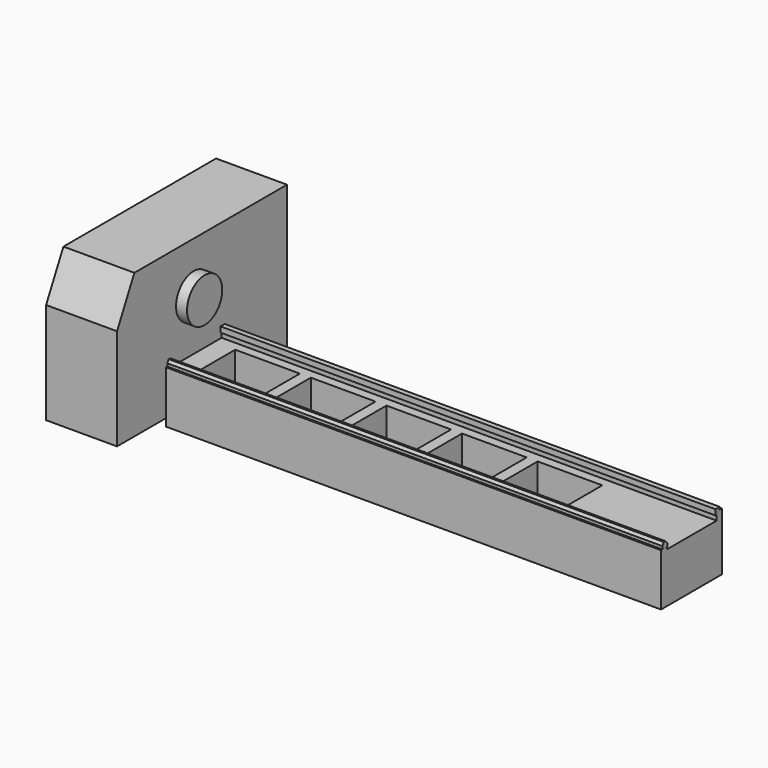
from build123d import *

# Parameters (mm, degrees)
F0_R     = 20
F1_DEPTH = 64.5
F0_W     = 69.1690184176
F0_H     = 6.8107743772
F2_DEPTH = 450
F3_W     = 402.7799852192
F3_H     = 51.0824993253
F4_DEPTH = 15
F5_W     = 58.800008148
F5_H     = 40.4249988496
F6_DEPTH = 40
F7_DEPTH = 450
F8_DEPTH = 10


# Not quite as in the source:
# - a feature names something its author has since deleted; it is built from what else it names


with BuildPart() as f1:
    # F0 (on Right) → F1 (new body)
    with BuildSketch(Plane.YZ):
        Polygon((-87.0358720422, 23.9922005967), (-87.0358720422, -68.190318747), (-31.3871668349, -68.190318747), (-31.3871668349, -27.5489028139), (-29.7969614784, -27.5489028139), (-29.7969614784, -24.9276731835), (-28.2796746202, -22.2527954323), (-26.482412375, -22.2527954323), (-24.0200519564, -24.9276731835), (-24.0200519564, -27.412929792), (-24.6065106683, -27.412929792), (-24.6065106683, -29.5631634037), (31.7927369408, -29.5631634037), (31.7927369408, -24.8985635082), (30.5205726556, -24.8985635082), (30.5205726556, -19.9159244041), (35.2954028477, -19.9159244041), (35.2954028477, -22.2527954323), (37.7818515827, -22.2527954323), (37.7818515827, -68.190318747), (106.1147302389, -68.190318747), (106.1147302389, 62.7493981556), (-67.339591682, 62.7493981556), align=None)
        with Locations((0, 16.7493981556)):
            Circle(F0_R, mode=Mode.SUBTRACT)
        Polygon((-31.3871668349, -27.5489028139), (-31.3871668349, -68.190318747), (37.7818515827, -68.190318747), (37.7818515827, -22.2527954323), (35.2954028477, -22.2527954323), (31.7927369408, -24.8985635082), (31.7927369408, -29.5631634037), (-24.6065106683, -29.5631634037), (-24.6065106683, -27.412929792), (-29.7969614784, -27.5489028139), align=None)
        with Locations((0, 16.7493981556)):
            Circle(F0_R)
        Polygon((-29.7969614784, -24.9276731835), (-29.7969614784, -27.5489028139), (-24.6065106683, -27.412929792), (-24.0200519564, -27.412929792), (-24.0200519564, -24.9276731835), (-26.482412375, -22.2527954323), (-28.2796746202, -22.2527954323), align=None)
        Polygon((31.7927369408, -24.8985635082), (35.2954028477, -22.2527954323), (35.2954028477, -19.9159244041), (30.5205726556, -19.9159244041), (30.5205726556, -24.8985635082), align=None)
    extrude(amount=-F1_DEPTH)


with BuildPart() as f2:
    # F0 (on Right) → F2 (new body)
    with BuildSketch(Plane.YZ):
        with Locations((3.1973423739, -71.5957059356)):
            Rectangle(F0_W, F0_H)
        Polygon((-31.3871668349, -27.5489028139), (-31.3871668349, -68.190318747), (37.7818515827, -68.190318747), (37.7818515827, -22.2527954323), (35.2954028477, -22.2527954323), (31.7927369408, -24.8985635082), (31.7927369408, -29.5631634037), (-24.6065106683, -29.5631634037), (-24.6065106683, -27.412929792), (-29.7969614784, -27.5489028139), align=None)
    extrude(amount=F2_DEPTH)

    # F3 (on face) → F4 (cut)
    with BuildSketch(Plane(origin=(0, 0, -75.0010931242), x_dir=(1, 0, 0), z_dir=(0, 0, -1))):
        with Locations((225.1687403768, -2.7406793088)):
            Rectangle(F3_W, F3_H)
    extrude(amount=-F4_DEPTH, mode=Mode.SUBTRACT)

    # F5 (on face) → F6 (cut)
    with BuildSketch(Plane.XY.offset(-29.5631634037)):
        with Locations((48.4012458473, 3.2919291407)):
            Rectangle(F5_W, F5_H)
        with Locations((323.291266337, 3.2919291407)):
            Rectangle(F5_W, F5_H)
        with Locations((117.1237509698, 3.2919291407)):
            Rectangle(F5_W, F5_H)
        with Locations((185.8462560922, 3.2919291407)):
            Rectangle(F5_W, F5_H)
        with Locations((254.5687612146, 3.2919291407)):
            Rectangle(F5_W, F5_H)
    extrude(amount=-F6_DEPTH, mode=Mode.SUBTRACT)


with BuildPart() as f7:
    # F0 (on Right) → F7 (new body)
    with BuildSketch(Plane.YZ):
        Polygon((-29.7969614784, -24.9276731835), (-29.7969614784, -27.5489028139), (-24.6065106683, -27.412929792), (-24.0200519564, -27.412929792), (-24.0200519564, -24.9276731835), (-26.482412375, -22.2527954323), (-28.2796746202, -22.2527954323), align=None)
    extrude(amount=F7_DEPTH)


with BuildPart() as f7b:
    # F0 (on Right) → F7, piece 2 (new body)
    with BuildSketch(Plane.YZ):
        Polygon((31.7927369408, -24.8985635082), (35.2954028477, -22.2527954323), (35.2954028477, -19.9159244041), (30.5205726556, -19.9159244041), (30.5205726556, -24.8985635082), align=None)
    extrude(amount=F7_DEPTH)


with BuildPart() as f8:
    # F0 (on Right) → F8 (new body)
    with BuildSketch(Plane.YZ):
        with Locations((0, 16.7493981556)):
            Circle(F0_R)
    extrude(amount=F8_DEPTH)


solid = Compound([f1.part, f2.part, f7.part, f7b.part, f8.part])
